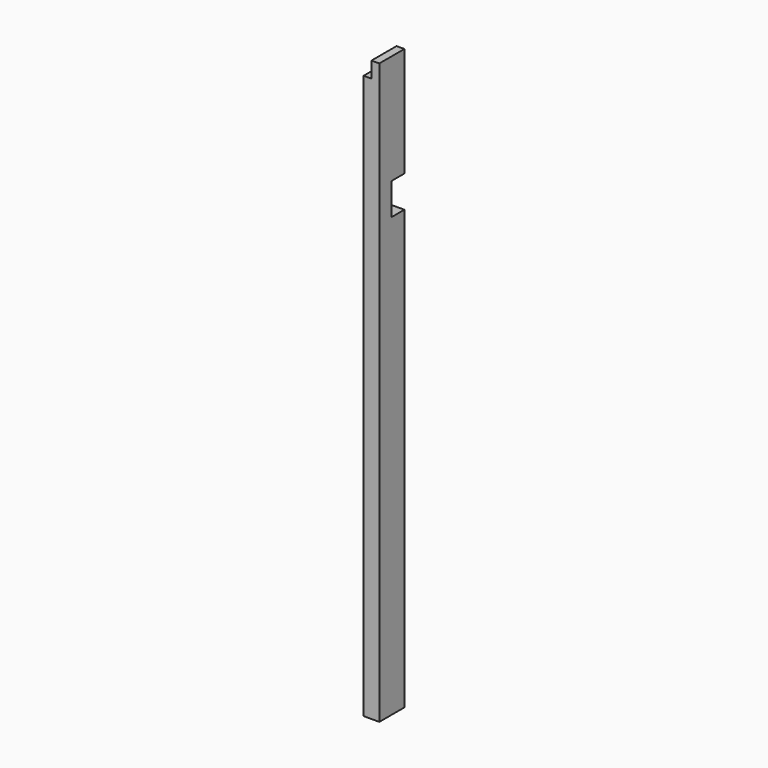
from build123d import *

# Parameters (mm, degrees)
F0_W     = 50
F0_H     = 100
F1_DEPTH = 1850
F2_W     = 50.8
F2_H     = 101.6
F3_DEPTH = 50
F4_W     = 25
F4_H     = 100
F5_DEPTH = 50.8


# Not quite as in the source:
# - a feature names something its author has since deleted; it is built from what else it names


with BuildPart() as f1:
    # F0 (on Top) → F1 (new body)
    with BuildSketch(Plane.XY):
        Rectangle(F0_W, F0_H)
    extrude(amount=F1_DEPTH)

    # F2 (on Right) → F3 (cut, symmetric)
    with BuildSketch(Plane.YZ):
        with Locations((24.6, 1449.2)):
            Rectangle(F2_W, F2_H)
    extrude(amount=F3_DEPTH, both=True, mode=Mode.SUBTRACT)

    # F4 (on face) → F5 (cut)
    with BuildSketch(Plane.XY.offset(1850)):
        with Locations((-12.5, 0)):
            Rectangle(F4_W, F4_H)
    extrude(amount=-F5_DEPTH, mode=Mode.SUBTRACT)


solid = f1.part
